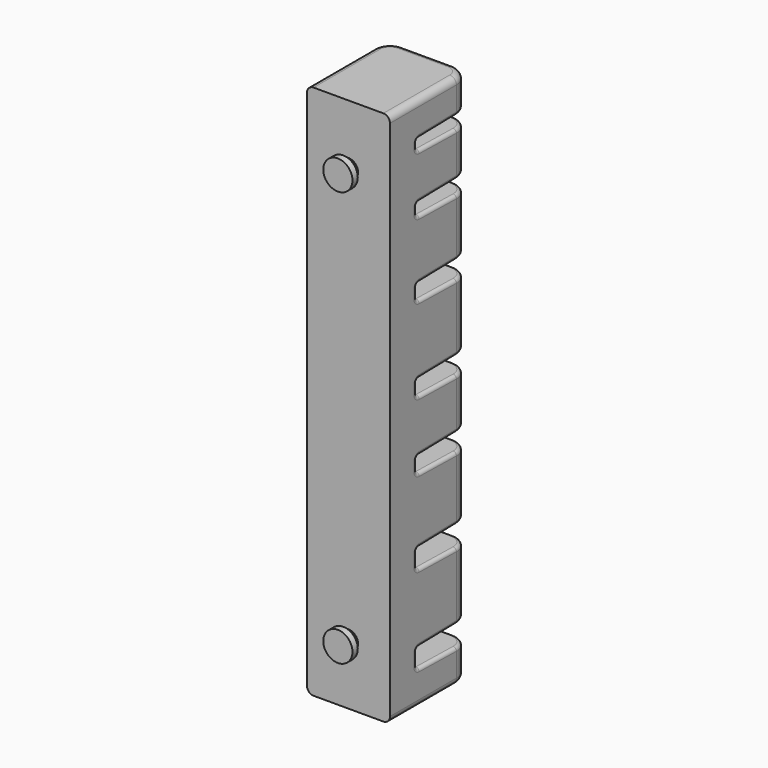
from build123d import *

# Parameters (mm, degrees)
F1_DEPTH = 25
F2_R     = 2.9
F3_DEPTH = 2
F4_R     = 4.4
F5_DEPTH = 2
F6_R     = 5
F7_R     = 2
F8_R     = 1
F9_R     = 1


# Not quite as in the source:
# - a feature names something its author has since deleted; it is built from what else it names


with BuildPart() as f1:
    # F0 (on Right) → F1 (new body)
    with BuildSketch(Plane.YZ):
        Polygon((-20, 15.9964008397), (0, 16.3964008397), (0, 36.3964008397), (-20, 36.7964008397), (-20, 42.3928016795), (0, 42.7928016795), (0, 61.7928016795), (-20, 62.1928016795), (-20, 66.7898023793), (0, 67.1898023793), (0, 82.1898023793), (-20, 82.5898023793), (-20, 87.186803079), (0, 87.586803079), (0, 107.586803079), (-20, 107.986803079), (-20, 112.5838037788), (0, 112.9838037788), (0, 129.9838037788), (-20, 130.3838037788), (-20, 133.9814043386), (0, 134.3814043386), (0, 147.3814043386), (-20, 147.7814043386), (-20, 150.8793048285), (0, 151.2793048285), (0, 161.2793048285), (-30, 161.2793048285), (-30, 0), (0, 0), (0, 10), (-20, 10.4), align=None)
    extrude(amount=F1_DEPTH)

    # F2 (on face) → F3 (join)
    with BuildSketch(Plane.XZ.offset(30)):
        with Locations((12.5, 143.1396524142)):
            Circle(F2_R)
        with Locations((12.5, 18.1396524142)):
            Circle(F2_R)
    extrude(amount=F3_DEPTH)

    # F4 (on face) → F5 (join)
    with BuildSketch(Plane.XZ.offset(32)):
        with Locations((12.5, 143.1396524142)):
            Circle(F4_R)
        with Locations((12.5, 18.1396524142)):
            Circle(F4_R)
    extrude(amount=F5_DEPTH)

    # F6
    f6_edges = [f1.edges().sort_by_distance(p)[0] for p in [
        (25, 0, 140.881404),
        (25, 0, 121.483804),
        (25, 0, 97.586803),
        (25, 0, 74.689802),
        (25, 0, 52.292802),
        (25, 0, 26.396401),
        (25, 0, 5),
        (0, 0, 140.881404),
        (0, 0, 121.483804),
        (0, 0, 97.586803),
        (0, 0, 74.689802),
        (0, 0, 52.292802),
        (0, 0, 26.396401),
        (0, 0, 5),
        (25, 0, 156.279305),
        (0, 0, 156.279305),
    ]]
    fillet(f6_edges, radius=F6_R)

    # F7
    f7_edges = [f1.edges().sort_by_distance(p)[0] for p in [
        (25, -17.5, 161.279305),
        (25, -17.5, 0),
    ]]
    fillet(f7_edges, radius=F7_R)

    # F8
    f8_edges = [f1.edges().sort_by_distance(p)[0] for p in [
        (12.5, -20, 15.996401),
        (12.5, -20, 42.392802),
        (12.5, -20, 66.789802),
        (12.5, -20, 87.186803),
        (12.5, -20, 112.583804),
        (12.5, -20, 133.981404),
        (12.5, -20, 150.879305),
        (12.5, -20, 10.4),
        (12.5, -20, 36.796401),
        (12.5, -20, 62.192802),
        (12.5, -20, 82.589802),
        (12.5, -20, 107.986803),
        (12.5, -20, 130.383804),
        (12.5, -20, 147.781404),
    ]]
    fillet(f8_edges, radius=F8_R)

    # F9
    f9_edges = [f1.edges().sort_by_distance(p)[0] for p in [
        (25, -12.009998, 147.621604),
        (25, -12.009998, 130.224004),
        (25, -12.009998, 107.827003),
        (25, -12.009998, 82.430002),
        (25, -12.009998, 62.033002),
        (25, -12.009998, 36.636601),
        (25, -12.009998, 10.2402),
    ]]
    fillet(f9_edges, radius=F9_R)


solid = f1.part
